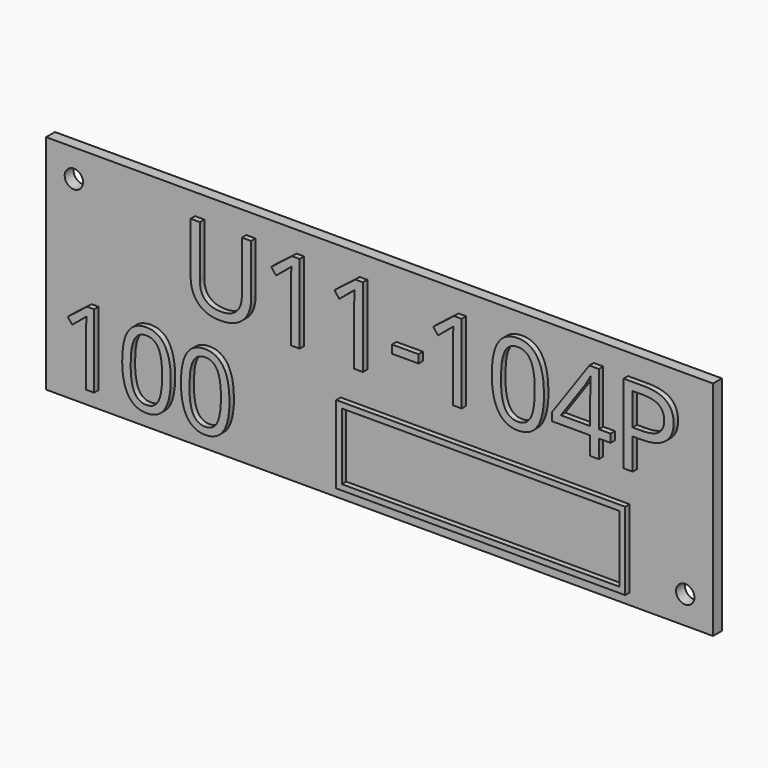
from build123d import *

# Parameters (mm, degrees)
F0_W         = 120
F0_H         = 40
F1_DEPTH     = 2
F3_D         = 3.3
F4_TEXT_SIZE = 19.8943114703
F5_DEPTH     = 1
F6_TEXT_SIZE = 18.4937691891
F7_DEPTH     = 1
F8_W         = 52
F8_H         = 14
F8_W_2       = 49.99999962
F8_H_2       = 11.99999962
F9_DEPTH     = 1


# Not quite as in the source:
# - Text() gives the source's letters only with a copy of the font that has no kerning and outlines rounded to 1/6400 em; it was checked with that copy


with BuildPart() as f1:
    # F0 (on Front) → F1 (new body)
    with BuildSketch(Plane.XZ):
        Rectangle(F0_W, F0_H)
    extrude(amount=F1_DEPTH)

    # F3 (through all)
    with Locations(Plane.XZ.offset(2)):
        with Locations((-55, 15), (55, -15)):
            Hole(F3_D / 2)

    # F4 (on face) → F5 (join)
    with BuildSketch(Plane.XZ.offset(2)):
        with Locations((-35, 2)):
            Text('U11-104P', F4_TEXT_SIZE, font='Open Sans', text_align=(TextAlign.LEFT, TextAlign.BOTTOM))
    extrude(amount=F5_DEPTH)

    # F6 (on face) → F7 (join)
    with BuildSketch(Plane.XZ.offset(2)):
        with Locations((-57, -17)):
            Text('100', F6_TEXT_SIZE, font='Open Sans', text_align=(TextAlign.LEFT, TextAlign.BOTTOM))
    extrude(amount=F7_DEPTH)

    # F8 (on face) → F9 (join)
    with BuildSketch(Plane.XZ.offset(2)):
        with Locations((19, -11)):
            Rectangle(F8_W, F8_H)
        with Locations((19, -11)):
            Rectangle(F8_W_2, F8_H_2, mode=Mode.SUBTRACT)
    extrude(amount=F9_DEPTH)


solid = f1.part
